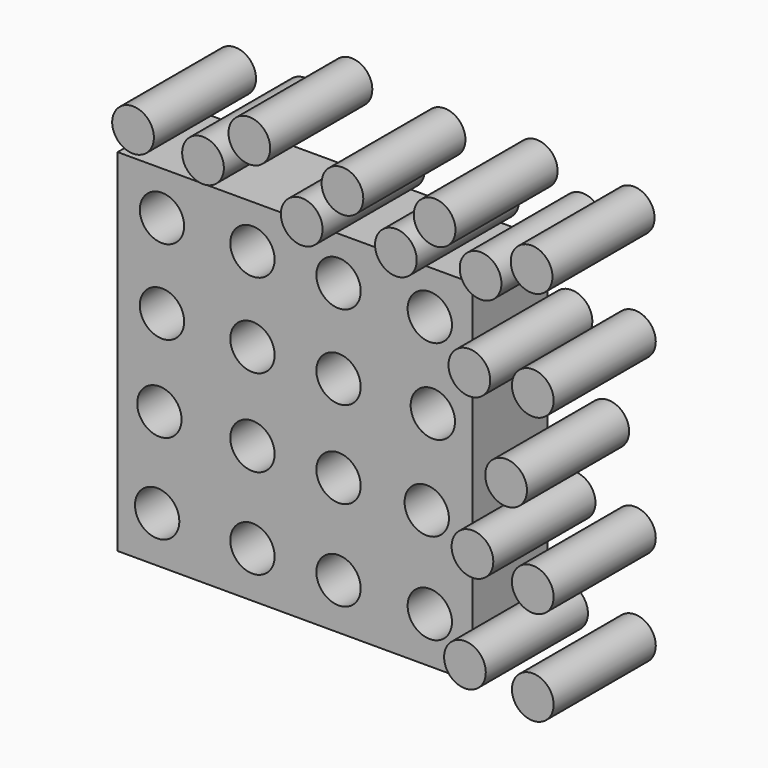
from build123d import *

# Parameters (mm, degrees)
F0_W     = 26.4658074026
F0_H     = 25.4
F0_R     = 6.6164518507
F0_H_2   = 26.4658074026
F1_DEPTH = 25.4
F2_W     = 105.8632296105
F2_H     = 104.7974222079
F3_DEPTH = 2.54
F4_R     = 6.223
F5_DEPTH = 38.1


# Not quite as in the source:
# - a feature names something its author has since deleted; it is built from what else it names


with BuildPart() as f1:
    # F0 (on Front) → F1 (new body)
    with BuildSketch(Plane.XZ):
        with Locations((-59.7954421587, 33.5575119803)):
            Rectangle(F0_W, F0_H)
        with Locations((-59.7954421587, 33.2744792104)):
            Circle(F0_R, mode=Mode.SUBTRACT)
        with Locations((19.6019800492, 33.5575119803)):
            Rectangle(F0_W, F0_H)
        with Locations((20.1159380376, 33.2744792104)):
            Circle(F0_R, mode=Mode.SUBTRACT)
        with Locations((-59.7954421587, -45.3070065262)):
            Rectangle(F0_W, F0_H_2)
        with Locations((-61.233740398, -44.7741028249)):
            Circle(F0_R, mode=Mode.SUBTRACT)
        with Locations((19.6019800492, -45.3070065262)):
            Rectangle(F0_W, F0_H_2)
        with Locations((20.1159380376, -44.7741028249)):
            Circle(F0_R, mode=Mode.SUBTRACT)
        with Locations((-6.8638273535, 33.5575119803)):
            Rectangle(F0_W, F0_H)
        with Locations((-7.108640857, 33.2744792104)):
            Circle(F0_R, mode=Mode.SUBTRACT)
        with Locations((-33.3296347561, -45.3070065262)):
            Rectangle(F0_W, F0_H_2)
        with Locations((-32.7967310548, -44.7741028249)):
            Circle(F0_R, mode=Mode.SUBTRACT)
        with Locations((-6.8638273535, -45.3070065262)):
            Rectangle(F0_W, F0_H_2)
        with Locations((-7.108640857, -44.7741028249)):
            Circle(F0_R, mode=Mode.SUBTRACT)
        with Locations((-59.7954421587, 7.624608279)):
            Rectangle(F0_W, F0_H_2)
        with Locations((-59.7954421587, 8.1575119803)):
            Circle(F0_R, mode=Mode.SUBTRACT)
        with Locations((-59.7954421587, -18.8411991236)):
            Rectangle(F0_W, F0_H_2)
        with Locations((-60.5651258442, -17.8472213447)):
            Circle(F0_R, mode=Mode.SUBTRACT)
        with Locations((19.6019800492, 7.624608279)):
            Rectangle(F0_W, F0_H_2)
        with Locations((21.0234187543, 8.1575119803)):
            Circle(F0_R, mode=Mode.SUBTRACT)
        with Locations((19.6019800492, -18.8411991236)):
            Rectangle(F0_W, F0_H_2)
        with Locations((19.208451733, -17.8472213447)):
            Circle(F0_R, mode=Mode.SUBTRACT)
        with Locations((-33.3296347561, 7.624608279)):
            Rectangle(F0_W, F0_H_2)
        with Locations((-32.7967310548, 8.1575119803)):
            Circle(F0_R, mode=Mode.SUBTRACT)
        with Locations((-6.8638273535, 7.624608279)):
            Rectangle(F0_W, F0_H_2)
        with Locations((-7.108640857, 8.1575119803)):
            Circle(F0_R, mode=Mode.SUBTRACT)
        with Locations((-6.8638273535, -18.8411991236)):
            Rectangle(F0_W, F0_H_2)
        with Locations((-7.108640857, -17.8472213447)):
            Circle(F0_R, mode=Mode.SUBTRACT)
        with Locations((-33.3296347561, -18.8411991236)):
            Rectangle(F0_W, F0_H_2)
        with Locations((-32.7967310548, -17.8472213447)):
            Circle(F0_R, mode=Mode.SUBTRACT)
        with Locations((-33.3296347561, 33.5575119803)):
            Rectangle(F0_W, F0_H)
        with Locations((-32.7967310548, 33.2744792104)):
            Circle(F0_R, mode=Mode.SUBTRACT)
    extrude(amount=F1_DEPTH)

    # F2 (on face) → F3 (join)
    with BuildSketch(Plane(origin=(0, 0, 0), x_dir=(-1, 0, 0), z_dir=(0, 1, 0))):
        with Locations((20.0967310548, -6.1411991236)):
            Rectangle(F2_W, F2_H)
    extrude(amount=F3_DEPTH)


with BuildPart() as f5:
    # F4 (on Front) → F5 (new body)
    with BuildSketch(Plane.XZ):
        with Locations((-58.2731813192, 62.0402358472)):
            Circle(F4_R)
    extrude(amount=F5_DEPTH)


with BuildPart() as f5b:
    # F4 (on Front) → F5, piece 2 (new body)
    with BuildSketch(Plane.XZ):
        with Locations((-37.3917855322, 60.8228035271)):
            Circle(F4_R)
    extrude(amount=F5_DEPTH)


with BuildPart() as f5c:
    # F4 (on Front) → F5, piece 3 (new body)
    with BuildSketch(Plane.XZ):
        with Locations((-23.5726330429, 70.5089494586)):
            Circle(F4_R)
    extrude(amount=F5_DEPTH)


with BuildPart() as f5d:
    # F4 (on Front) → F5, piece 4 (new body)
    with BuildSketch(Plane.XZ):
        with Locations((-7.9380692914, 54.2975701392)):
            Circle(F4_R)
    extrude(amount=F5_DEPTH)


with BuildPart() as f5e:
    # F4 (on Front) → F5, piece 5 (new body)
    with BuildSketch(Plane.XZ):
        with Locations((4.2139817961, 66.332988441)):
            Circle(F4_R)
    extrude(amount=F5_DEPTH)


with BuildPart() as f5f:
    # F4 (on Front) → F5, piece 6 (new body)
    with BuildSketch(Plane.XZ):
        with Locations((20.1564356685, 55.3406402469)):
            Circle(F4_R)
    extrude(amount=F5_DEPTH)


with BuildPart() as f5g:
    # F4 (on Front) → F5, piece 7 (new body)
    with BuildSketch(Plane.XZ):
        with Locations((31.7162796855, 67.0352354646)):
            Circle(F4_R)
    extrude(amount=F5_DEPTH)


with BuildPart() as f5h:
    # F4 (on Front) → F5, piece 8 (new body)
    with BuildSketch(Plane.XZ):
        with Locations((45.4349666834, 57.44157359)):
            Circle(F4_R)
    extrude(amount=F5_DEPTH)


with BuildPart() as f5i:
    # F4 (on Front) → F5, piece 9 (new body)
    with BuildSketch(Plane.XZ):
        with Locations((60.6517754495, 64.150698483)):
            Circle(F4_R)
    extrude(amount=F5_DEPTH)


with BuildPart() as f5j:
    # F4 (on Front) → F5, piece 10 (new body)
    with BuildSketch(Plane.XZ):
        with Locations((42.0833453536, 30.9337414801)):
            Circle(F4_R)
    extrude(amount=F5_DEPTH)


with BuildPart() as f5k:
    # F4 (on Front) → F5, piece 11 (new body)
    with BuildSketch(Plane.XZ):
        with Locations((61.0104165971, 31.7427292466)):
            Circle(F4_R)
    extrude(amount=F5_DEPTH)


with BuildPart() as f5l:
    # F4 (on Front) → F5, piece 12 (new body)
    with BuildSketch(Plane.XZ):
        with Locations((53.0484132469, 5.575186573)):
            Circle(F4_R)
    extrude(amount=F5_DEPTH)


with BuildPart() as f5m:
    # F4 (on Front) → F5, piece 13 (new body)
    with BuildSketch(Plane.XZ):
        with Locations((43.0077053607, -16.4317153394)):
            Circle(F4_R)
    extrude(amount=F5_DEPTH)


with BuildPart() as f5n:
    # F4 (on Front) → F5, piece 14 (new body)
    with BuildSketch(Plane.XZ):
        with Locations((61.0104165971, -19.8372639716)):
            Circle(F4_R)
    extrude(amount=F5_DEPTH)


with BuildPart() as f5o:
    # F4 (on Front) → F5, piece 15 (new body)
    with BuildSketch(Plane.XZ):
        with Locations((40.7665111125, -46.2394170463)):
            Circle(F4_R)
    extrude(amount=F5_DEPTH)


with BuildPart() as f5p:
    # F4 (on Front) → F5, piece 16 (new body)
    with BuildSketch(Plane.XZ):
        with Locations((61.0104165971, -48.1384880841)):
            Circle(F4_R)
    extrude(amount=F5_DEPTH)


solid = Compound([f1.part, f5.part, f5b.part, f5c.part, f5d.part, f5e.part, f5f.part, f5g.part, f5h.part, f5i.part, f5j.part, f5k.part, f5l.part, f5m.part, f5n.part, f5o.part, f5p.part])
